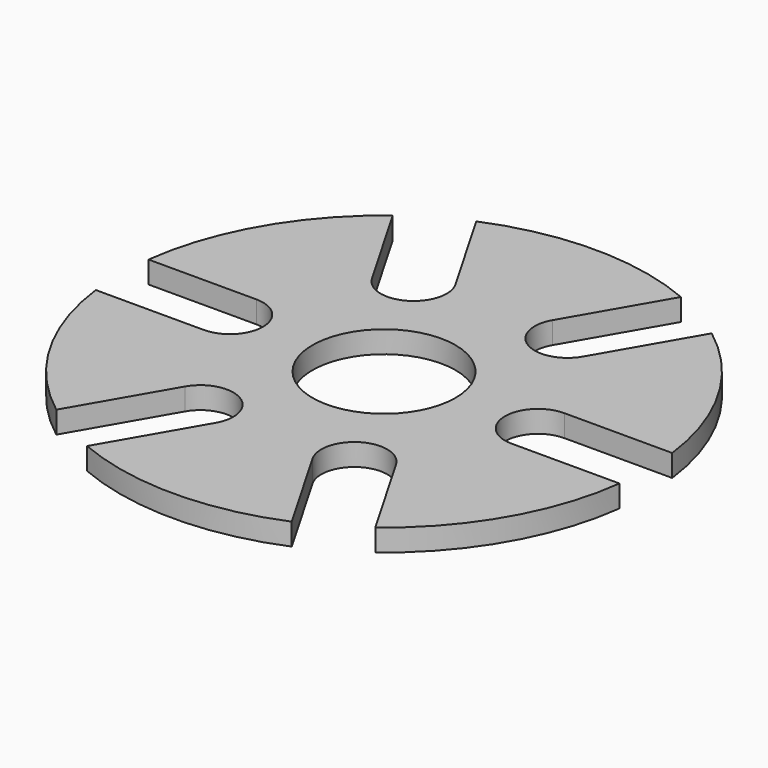
from build123d import *

# Parameters (mm, degrees)
F0_R     = 20.6375
F1_DEPTH = 6.35


# Not quite as in the source:
# - a feature names something its author has since deleted; it is built from what else it names


with BuildPart() as f1:
    # F0 (on Top) → F1 (new body)
    with BuildSketch(Plane.XY):
        with BuildLine():
            Line((-44.45, -9.525), (-75.6023437137, -9.525))
            ThreePointArc((-75.6023437137, -9.525), (-65.9911357684, -38.1), (-46.0500638279, -60.7110502417))
            Line((-46.0500638279, -60.7110502417), (-30.473891971, -33.7323291982))
            ThreePointArc((-30.473891971, -33.7323291982), (-17.4625, -30.2459372272), (-13.976108029, -43.2573291982))
            Line((-13.976108029, -43.2573291982), (-29.5522798858, -70.2360502417))
            ThreePointArc((-29.5522798858, -70.2360502417), (0, -76.2), (29.5522798858, -70.2360502417))
            Line((29.5522798858, -70.2360502417), (13.976108029, -43.2573291982))
            ThreePointArc((13.976108029, -43.2573291982), (17.4625, -30.2459372272), (30.473891971, -33.7323291982))
            Line((30.473891971, -33.7323291982), (46.0500638279, -60.7110502417))
            ThreePointArc((46.0500638279, -60.7110502417), (65.9911357684, -38.1), (75.6023437137, -9.525))
            Line((75.6023437137, -9.525), (44.45, -9.525))
            ThreePointArc((44.45, -9.525), (34.925, 0), (44.45, 9.525))
            Line((44.45, 9.525), (75.6023437137, 9.525))
            ThreePointArc((75.6023437137, 9.525), (65.9911357684, 38.1), (46.0500638279, 60.7110502417))
            Line((46.0500638279, 60.7110502417), (30.473891971, 33.7323291982))
            ThreePointArc((30.473891971, 33.7323291982), (17.4625, 30.2459372272), (13.976108029, 43.2573291982))
            Line((13.976108029, 43.2573291982), (29.5522798858, 70.2360502417))
            ThreePointArc((29.5522798858, 70.2360502417), (0, 76.2), (-29.5522798858, 70.2360502417))
            Line((-29.5522798858, 70.2360502417), (-13.976108029, 43.2573291982))
            ThreePointArc((-13.976108029, 43.2573291982), (-17.4625, 30.2459372272), (-30.473891971, 33.7323291982))
            Line((-30.473891971, 33.7323291982), (-46.0500638279, 60.7110502417))
            ThreePointArc((-46.0500638279, 60.7110502417), (-65.9911357684, 38.1), (-75.6023437137, 9.525))
            Line((-75.6023437137, 9.525), (-44.45, 9.525))
            ThreePointArc((-44.45, 9.525), (-34.925, 0), (-44.45, -9.525))
        make_face()
        Circle(F0_R, mode=Mode.SUBTRACT)
    extrude(amount=F1_DEPTH)


solid = f1.part
